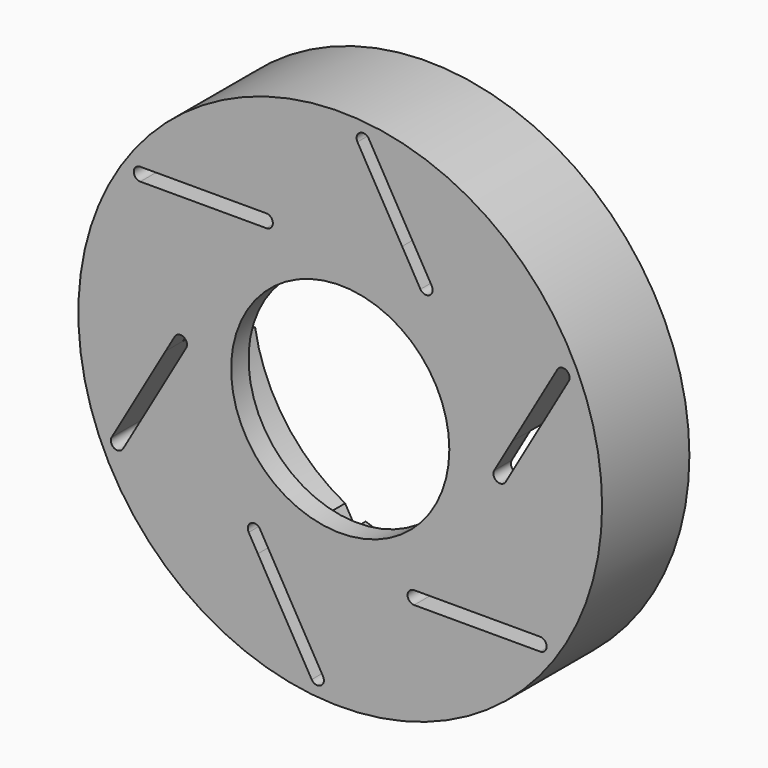
from build123d import *

# Parameters (mm, degrees)
F0_R     = 31.75
F1_DEPTH = 6.35
F0_R_2   = 76.2
F0_R_3   = 74.4988936807
F2_DEPTH = 31.75


# Not quite as in the source:
# - a feature names something its author has since deleted; it is built from what else it names


with BuildPart() as f1:
    # F0 (on Front) → F1 (new body)
    with BuildSketch(Plane.XZ):
        with BuildLine():
            ThreePointArc((47.0428302523, -32.9697150499), (60.8100722022, -15.3863528649), (65.7145588579, 6.4002849501))
            ThreePointArc((65.7145588579, 6.4002849501), (65.7078231144, 7.227857987), (65.6876176686, 8.0552117454))
            Line((65.6876176686, 8.0552117454), (63.0200884494, 3.4349156071))
            ThreePointArc((63.0200884494, 3.4349156071), (60.4178100552, 2.7376372129), (59.720531661, 5.3399156071))
            Line((59.720531661, 5.3399156071), (65.0529232684, 14.5758887971))
            ThreePointArc((65.0529232684, 14.5758887971), (56.2331130755, 35.9675096944), (38.8466881833, 51.2352117455))
            Line((38.8466881833, 51.2352117455), (41.5142174026, 46.6149156071))
            ThreePointArc((41.5142174026, 46.6149156071), (40.8169390084, 44.0126372129), (38.2146606142, 44.7099156071))
            Line((38.2146606142, 44.7099156071), (32.8822690066, 53.9458887971))
            ThreePointArc((32.8822690066, 53.9458887971), (9.9466767851, 57.0035195621), (-11.9687534946, 49.5802849501))
            Line((-11.9687534946, 49.5802849501), (-6.6336950562, 49.5802849501))
            ThreePointArc((-6.6336950562, 49.5802849501), (-4.7286950562, 47.6752849501), (-6.6336950562, 45.7702849501))
            Line((-6.6336950562, 45.7702849501), (-17.2984782711, 45.7702849501))
            ThreePointArc((-17.2984782711, 45.7702849501), (-31.4142602999, 27.4362948179), (-35.9432656874, 4.7453581548))
            Line((-35.9432656874, 4.7453581548), (-33.2757364682, 9.3656542931))
            ThreePointArc((-33.2757364682, 9.3656542931), (-30.673458074, 10.0629326873), (-29.9761796798, 7.4606542931))
            Line((-29.9761796798, 7.4606542931), (-35.3085712873, -1.7753188969))
            ThreePointArc((-35.3085712873, -1.7753188969), (-26.4887610944, -23.1669397942), (-9.1023362022, -38.4346418453))
            Line((-9.1023362022, -38.4346418453), (-11.7698654214, -33.8143457069))
            ThreePointArc((-11.7698654214, -33.8143457069), (-11.0725870272, -31.2120673127), (-8.470308633, -31.9093457069))
            Line((-8.470308633, -31.9093457069), (-3.1379170255, -41.1453188969))
            ThreePointArc((-3.1379170255, -41.1453188969), (19.797675196, -44.202949662), (41.7131054758, -36.7797150499))
            Line((41.7131054758, -36.7797150499), (36.3780470374, -36.7797150499))
            ThreePointArc((36.3780470374, -36.7797150499), (34.4730470374, -34.8747150499), (36.3780470374, -32.9697150499))
            Line((36.3780470374, -32.9697150499), (47.0428302523, -32.9697150499))
        make_face()
        with Locations((14.8721759906, 6.4002849501)):
            Circle(F0_R, mode=Mode.SUBTRACT)
    extrude(amount=-F1_DEPTH)

    # F0 (on Front) → F2 (join)
    with BuildSketch(Plane.XZ):
        with Locations((14.8721759906, 6.4002849501)):
            Circle(F0_R_2)
        with Locations((14.8721759906, 6.4002849501)):
            Circle(F0_R_3, mode=Mode.SUBTRACT)
        with Locations((14.8721759906, 6.4002849501)):
            Circle(F0_R_3)
        with BuildLine():
            ThreePointArc((65.6876176686, 8.0552117454), (65.7078231144, 7.227857987), (65.7145588579, 6.4002849501))
            ThreePointArc((65.7145588579, 6.4002849501), (60.8100722022, -15.3863528649), (47.0428302523, -32.9697150499))
            Line((47.0428302523, -32.9697150499), (73.0397974374, -32.9697150499))
            ThreePointArc((73.0397974374, -32.9697150499), (74.9447974374, -34.8747150499), (73.0397974374, -36.7797150499))
            Line((73.0397974374, -36.7797150499), (41.7131054758, -36.7797150499))
            ThreePointArc((41.7131054758, -36.7797150499), (19.797675196, -44.202949662), (-3.1379170255, -41.1453188969))
            Line((-3.1379170255, -41.1453188969), (9.860566567, -63.6593529005))
            ThreePointArc((9.860566567, -63.6593529005), (9.1632881728, -66.2616312948), (6.5610097786, -65.5643529005))
            Line((6.5610097786, -65.5643529005), (-9.1023362022, -38.4346418453))
            ThreePointArc((-9.1023362022, -38.4346418453), (-26.4887610944, -23.1669397942), (-35.3085712873, -1.7753188969))
            Line((-35.3085712873, -1.7753188969), (-48.3070548798, -24.2893529005))
            ThreePointArc((-48.3070548798, -24.2893529005), (-50.909333274, -24.9866312948), (-51.6066116682, -22.3843529005))
            Line((-51.6066116682, -22.3843529005), (-35.9432656874, 4.7453581548))
            ThreePointArc((-35.9432656874, 4.7453581548), (-31.4142602999, 27.4362948179), (-17.2984782711, 45.7702849501))
            Line((-17.2984782711, 45.7702849501), (-43.2954454562, 45.7702849501))
            ThreePointArc((-43.2954454562, 45.7702849501), (-45.2004454562, 47.6752849501), (-43.2954454562, 49.5802849501))
            Line((-43.2954454562, 49.5802849501), (-11.9687534946, 49.5802849501))
            ThreePointArc((-11.9687534946, 49.5802849501), (9.9466767851, 57.0035195621), (32.8822690066, 53.9458887971))
            Line((32.8822690066, 53.9458887971), (19.8837854141, 76.4599228007))
            ThreePointArc((19.8837854141, 76.4599228007), (20.5810638083, 79.0622011949), (23.1833422025, 78.3649228007))
            Line((23.1833422025, 78.3649228007), (38.8466881833, 51.2352117455))
            ThreePointArc((38.8466881833, 51.2352117455), (56.2331130755, 35.9675096944), (65.0529232684, 14.5758887971))
            Line((65.0529232684, 14.5758887971), (78.051406861, 37.0899228007))
            ThreePointArc((78.051406861, 37.0899228007), (80.6536852552, 37.7872011949), (81.3509636494, 35.1849228007))
            Line((81.3509636494, 35.1849228007), (65.6876176686, 8.0552117454))
        make_face(mode=Mode.SUBTRACT)
    extrude(amount=-F2_DEPTH)


solid = f1.part
